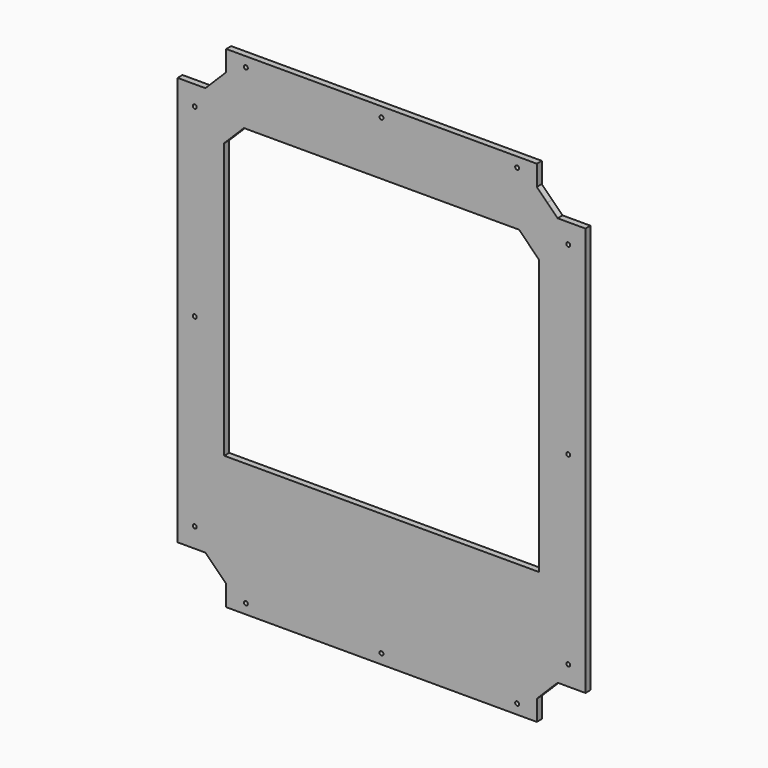
from build123d import *

# Parameters (mm, degrees)
F0_R     = 2.01
F1_DEPTH = 6.35


# Not quite as in the source:
# - a feature names something its author has since deleted; it is built from what else it names


with BuildPart() as f1:
    # F0 (on Front) → F1 (new body)
    with BuildSketch(Plane.XZ):
        Polygon((158, -229.1715728753), (168.5857864376, -218.5857864376), (179.1715728753, -208), (207.5215728753, -208), (207.5215728753, 208), (179.1715728753, 208), (168.5857864376, 218.5857864376), (158, 229.1715728753), (158, 240), (158, 250), (-158, 250), (-158, 240), (-158, 229.1715728753), (-168.5857864376, 218.5857864376), (-179.1715728753, 208), (-207.5215728753, 208), (-207.5215728753, -208), (-179.1715728753, -208), (-168.5857864376, -218.5857864376), (-158, -229.1715728753), (-158, -240), (-158, -250), (158, -250), (158, -240), align=None)
        with Locations((-190, -188)):
            Circle(F0_R, mode=Mode.SUBTRACT)
        with Locations((-138, -240)):
            Circle(F0_R, mode=Mode.SUBTRACT)
        with Locations((0, -240)):
            Circle(F0_R, mode=Mode.SUBTRACT)
        with Locations((138, -240)):
            Circle(F0_R, mode=Mode.SUBTRACT)
        with Locations((190, -188)):
            Circle(F0_R, mode=Mode.SUBTRACT)
        with Locations((-190, 0)):
            Circle(F0_R, mode=Mode.SUBTRACT)
        with Locations((-190, 188)):
            Circle(F0_R, mode=Mode.SUBTRACT)
        with Locations((-138, 240)):
            Circle(F0_R, mode=Mode.SUBTRACT)
        Polygon((-140, 185), (140, 185), (160, 165), (160, -115), (0, -115), (-160, -115), (-160, 165), align=None, mode=Mode.SUBTRACT)
        with Locations((190, 0)):
            Circle(F0_R, mode=Mode.SUBTRACT)
        with Locations((0, 240)):
            Circle(F0_R, mode=Mode.SUBTRACT)
        with Locations((138, 240)):
            Circle(F0_R, mode=Mode.SUBTRACT)
        with Locations((190, 188)):
            Circle(F0_R, mode=Mode.SUBTRACT)
    extrude(amount=F1_DEPTH)


solid = f1.part
